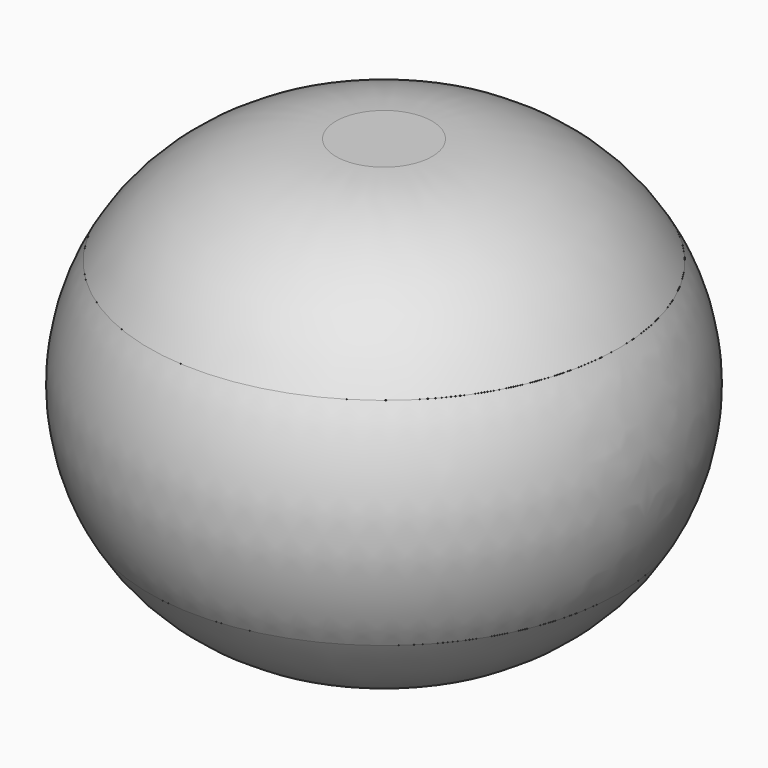
from build123d import *

# Parameters (mm, degrees)
F0_R      = 50.8
F1_DEPTH  = 63.5
F1_TAPER  = -30
F1_FACE_R = 87.4617420935
F2_DEPTH  = 63.5
F2_TAPER  = 30
F3_R      = 63.49999


# Not quite as in the source:
# - a fillet or chamfer is up to 0.001 mm smaller than in the source, because OpenCascade refuses the exact size


with BuildPart() as f1:
    # F0 (on Top) → F1 (new body)
    with BuildSketch(Plane.XY):
        Circle(F0_R)
    extrude(amount=F1_DEPTH, taper=F1_TAPER)

    # F1_face (on face) → F2 (join)
    with BuildSketch(Plane.XY.offset(63.5)):
        Circle(F1_FACE_R)
    extrude(amount=F2_DEPTH, taper=F2_TAPER)

    # F3 (radius 63.5 in the source; OpenCascade refuses exactly that, so slightly less here)
    f3_edges = [f1.edges().sort_by_distance(p)[0] for p in [
        (-87.461742, 0, 63.5),
        (-50.8, 0, 127),
        (-50.8, 0, 0),
    ]]
    fillet(f3_edges, radius=F3_R)


solid = f1.part
